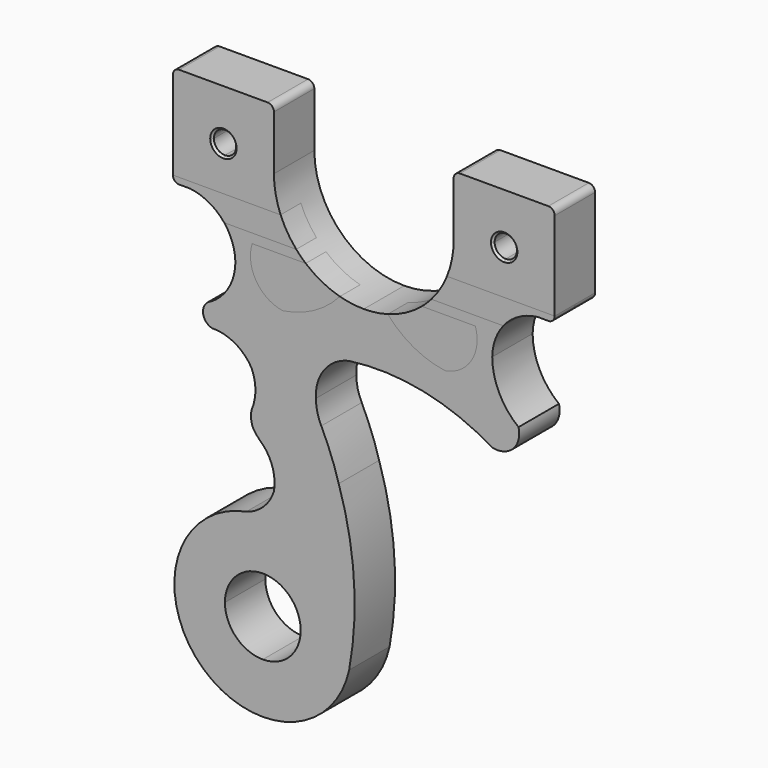
from build123d import *

# Parameters (mm, degrees)
F1_DEPTH = 12.7
F2_SIZE  = 0.508
F4_DEPTH = 6.35
F5_DEPTH = 6.35


with BuildPart() as f1:
    # F0 (on Front) → F1 (new body)
    with BuildSketch(Plane.XZ):
        with BuildLine():
            Line((-35.9628051519, 74.3345879376), (-35.9628051519, 52.1095879376))
            ThreePointArc((-35.9628051519, 52.1095879376), (-35.4978371671, 50.9870559225), (-34.3753051519, 50.5220879376))
            Line((-34.3753051519, 50.5220879376), (-31.7102633417, 50.5220879376))
            ThreePointArc((-31.7102633417, 50.5220879376), (-23.6045079295, 46.4058672096), (-20.2551409602, 37.9543416202))
            ThreePointArc((-20.2551409602, 37.9543416202), (-21.9138635475, 31.7764261625), (-26.4106839895, 27.2270739079))
            ThreePointArc((-26.4106839895, 27.2270739079), (-28.3924598426, 24.2357162237), (-26.1585302651, 21.4276537299))
            ThreePointArc((-26.1585302651, 21.4276537299), (-20.4079287218, 20.0003341812), (-16.1861311644, 15.8430412412))
            ThreePointArc((-16.1861311644, 15.8430412412), (-15.2200232553, 11.207539821), (-16.1861311644, 6.5720384009))
            ThreePointArc((-16.1861311644, 6.5720384009), (-16.3062460987, 4.5087014073), (-15.732049942, 2.5232327171))
            ThreePointArc((-15.732049942, 2.5232327171), (-14.5189102199, 0.951875362), (-13.1080421386, -0.4446643545))
            ThreePointArc((-13.1080421386, -0.4446643545), (-10.795687591, -4.7716751996), (-10.5683878064, -9.6725262702))
            ThreePointArc((-10.5683878064, -9.6725262702), (-13.1984563019, -13.8877028461), (-17.5003244607, -16.3734430181))
            ThreePointArc((-17.5003244607, -16.3734430181), (-29.3118646244, -53.699793422), (8.3489892293, -43.002644151))
            ThreePointArc((8.3489892293, -43.002644151), (9.557638386, -22.651764197), (5.7222023606, -2.6290626265))
            ThreePointArc((5.7222023606, -2.6290626265), (3.7814770492, 3.1455305799), (1.3426912483, 8.728062734))
            ThreePointArc((1.3426912483, 8.728062734), (0.3379920997, 11.4796705796), (0, 14.3894003704))
            ThreePointArc((0, 14.3894003704), (2.1128447305, 21.423665691), (8.2974387333, 25.3854580224))
            ThreePointArc((8.2974387333, 25.3854580224), (26.9445854097, 24.7346775815), (44.3060602993, 17.899563536))
            ThreePointArc((44.3060602993, 17.899563536), (47.2383051728, 17.9992305099), (49.741897732, 19.5289421827))
            ThreePointArc((49.741897732, 19.5289421827), (50.952066256, 21.9105950176), (50.9217604995, 24.5818980038))
            ThreePointArc((50.9217604995, 24.5818980038), (46.0830273259, 30.5107516192), (44.3060602993, 37.9543416202))
            ThreePointArc((44.3060602993, 37.9543416202), (47.6554272686, 46.4058672096), (55.7611826807, 50.5220879376))
            Line((55.7611826807, 50.5220879376), (58.426224491, 50.5220879376))
            ThreePointArc((58.426224491, 50.5220879376), (59.5487565061, 50.9870559225), (60.013724491, 52.1095879376))
            Line((60.013724491, 52.1095879376), (60.013724491, 74.3345879376))
            ThreePointArc((60.013724491, 74.3345879376), (59.5487565061, 75.4571199527), (58.426224491, 75.9220879376))
            Line((58.426224491, 75.9220879376), (36.201224491, 75.9220879376))
            ThreePointArc((36.201224491, 75.9220879376), (35.0786924759, 75.4571199527), (34.613724491, 74.3345879376))
            Line((34.613724491, 74.3345879376), (34.613724491, 60.6561478734))
            ThreePointArc((34.613724491, 60.6561478734), (27.9977749, 44.6838326429), (12.0254596695, 38.0678830519))
            ThreePointArc((12.0254596695, 38.0678830519), (-3.946855561, 44.6838326429), (-10.5628051519, 60.6561478734))
            Line((-10.5628051519, 60.6561478734), (-10.5628051519, 74.3345879376))
            ThreePointArc((-10.5628051519, 74.3345879376), (-11.0277731368, 75.4571199527), (-12.1503051519, 75.9220879376))
            Line((-12.1503051519, 75.9220879376), (-34.3753051519, 75.9220879376))
            ThreePointArc((-34.3753051519, 75.9220879376), (-35.4978371671, 75.4571199527), (-35.9628051519, 74.3345879376))
        make_face()
        with BuildLine():
            ThreePointArc((-13.3603820577, -28.6904807448), (-6.6251899669, -31.480288654), (-3.8353820577, -38.2154807448))
            ThreePointArc((-3.8353820577, -38.2154807448), (-6.6251899669, -44.9506728356), (-13.3603820577, -47.7404807448))
            ThreePointArc((-13.3603820577, -47.7404807448), (-20.0955741485, -44.9506728356), (-22.8853820577, -38.2154807448))
            ThreePointArc((-22.8853820577, -38.2154807448), (-20.0955741485, -31.480288654), (-13.3603820577, -28.6904807448))
        make_face(mode=Mode.SUBTRACT)
        with BuildLine():
            ThreePointArc((-20.4561051519, 63.2220879376), (-21.2781685492, 61.2374513348), (-23.2628051519, 60.4153879376))
            ThreePointArc((-23.2628051519, 60.4153879376), (-25.2474417547, 61.2374513348), (-26.0695051519, 63.2220879376))
            ThreePointArc((-26.0695051519, 63.2220879376), (-25.2474417547, 65.2067245403), (-23.2628051519, 66.0287879376))
            ThreePointArc((-23.2628051519, 66.0287879376), (-21.2781685492, 65.2067245403), (-20.4561051519, 63.2220879376))
        make_face(mode=Mode.SUBTRACT)
        with BuildLine():
            ThreePointArc((47.313724491, 66.0287879376), (49.2983610938, 65.2067245403), (50.120424491, 63.2220879376))
            ThreePointArc((50.120424491, 63.2220879376), (49.2983610938, 61.2374513348), (47.313724491, 60.4153879376))
            ThreePointArc((47.313724491, 60.4153879376), (45.3290878882, 61.2374513348), (44.507024491, 63.2220879376))
            ThreePointArc((44.507024491, 63.2220879376), (45.3290878882, 65.2067245403), (47.313724491, 66.0287879376))
        make_face(mode=Mode.SUBTRACT)
    extrude(amount=F1_DEPTH)

    # F2
    f2_edges = [f1.edges().sort_by_distance(p)[0] for p in [
        (-23.262805, -12.7, 60.415388),
        (47.313724, -12.7, 66.028788),
        (47.313724, 0, 66.028788),
        (-23.262805, 0, 60.415388),
    ]]
    chamfer(f2_edges, length=F2_SIZE)

    # F3 (on face) → F4 (cut)
    with BuildSketch(Plane.XZ.offset(12.7)):
        with BuildLine():
            Line((-8.8835341109, 52.1095879376), (-35.9628051519, 52.1095879376))
            ThreePointArc((-35.9628051519, 52.1095879376), (-35.4978371671, 50.9870559225), (-34.3753051519, 50.5220879376))
            Line((-34.3753051519, 50.5220879376), (-31.7102633417, 50.5220879376))
            ThreePointArc((-31.7102633417, 50.5220879376), (-26.9055008974, 49.0067085852), (-23.0534458939, 45.75958848))
            Line((-23.0534458939, 45.75958848), (-4.9545940961, 45.75958848))
            ThreePointArc((-4.9545940961, 45.75958848), (-7.1832780366, 48.7711109201), (-8.8835341109, 52.1095879376))
        make_face()
        with BuildLine():
            Line((60.013724491, 52.1095879376), (32.9344534499, 52.1095879376))
            ThreePointArc((32.9344534499, 52.1095879376), (31.2341973757, 48.7711109201), (29.0055134352, 45.75958848))
            Line((29.0055134352, 45.75958848), (47.104365233, 45.75958848))
            ThreePointArc((47.104365233, 45.75958848), (50.9564202365, 49.0067085852), (55.7611826807, 50.5220879376))
            Line((55.7611826807, 50.5220879376), (58.426224491, 50.5220879376))
            ThreePointArc((58.426224491, 50.5220879376), (59.5487565061, 50.9870559225), (60.013724491, 52.1095879376))
        make_face()
        with BuildLine():
            Line((40.0793049484, 43.4168316424), (26.6212016353, 43.4168316424))
            ThreePointArc((26.6212016353, 43.4168316424), (22.5799758765, 40.6853718424), (18.0465854352, 38.8851636936))
            ThreePointArc((18.0465854352, 38.8851636936), (24.5354070051, 33.6806648499), (32.4300676584, 31.0603696853))
            ThreePointArc((32.4300676584, 31.0603696853), (39.084946833, 35.4865348655), (40.0793049484, 43.4168316424))
        make_face()
        with BuildLine():
            ThreePointArc((6.0043339039, 38.8851636936), (1.4709434626, 40.6853718424), (-2.5702822963, 43.4168316424))
            Line((-2.5702822963, 43.4168316424), (-16.0283856094, 43.4168316424))
            ThreePointArc((-16.0283856094, 43.4168316424), (-15.0340274939, 35.4865348655), (-8.3791483194, 31.0603696853))
            ThreePointArc((-8.3791483194, 31.0603696853), (-0.4844876661, 33.6806648499), (6.0043339039, 38.8851636936))
        make_face()
    extrude(amount=-F4_DEPTH, mode=Mode.SUBTRACT)


with BuildPart() as f5:
    # F5 (new): a face of the model
    f5_faces = [f1.part.faces().sort_by_distance(p)[0] for p in [
        (-18.2506791882, -6.35, 49.2131238692),
    ]]
    extrude(f5_faces, amount=F5_DEPTH)


with BuildPart() as f5b:
    # F5#2 (new): a face of the model
    f5_2_faces = [f1.part.faces().sort_by_distance(p)[0] for p in [
        (42.3015985272, -6.35, 49.2131238692),
    ]]
    extrude(f5_2_faces, amount=F5_DEPTH)


with BuildPart() as f5c:
    # F5#3 (new): a face of the model
    f5_3_faces = [f1.part.faces().sort_by_distance(p)[0] for p in [
        (-6.7748141706, -6.35, 37.8823444138),
    ]]
    extrude(f5_3_faces, amount=F5_DEPTH)


with BuildPart() as f5d:
    # F5#4 (new): a face of the model
    f5_4_faces = [f1.part.faces().sort_by_distance(p)[0] for p in [
        (30.8257335097, -6.35, 37.8823444138),
    ]]
    extrude(f5_4_faces, amount=F5_DEPTH)


solid = Compound([f1.part, f5.part, f5b.part, f5c.part, f5d.part])
